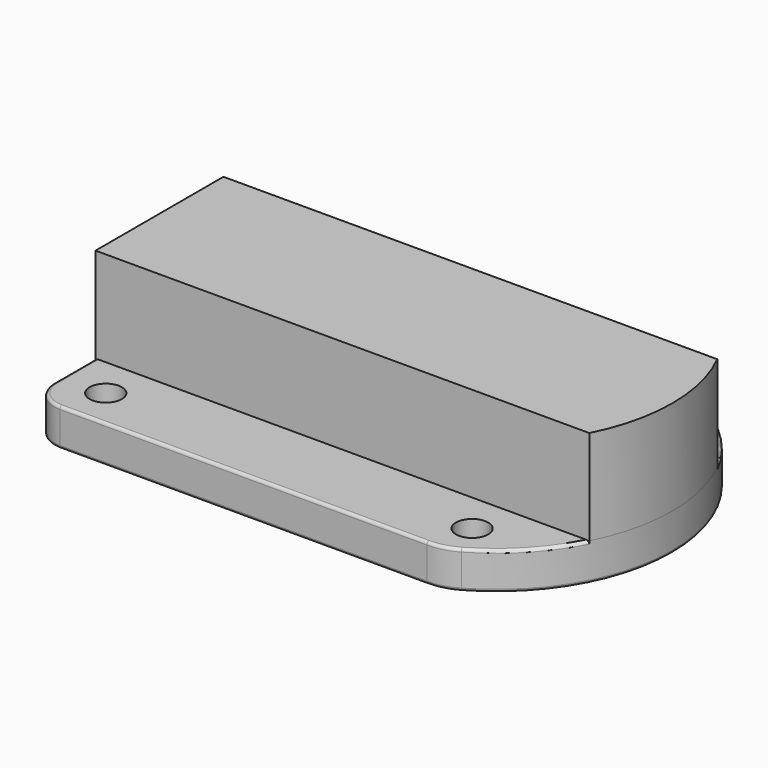
from build123d import *

# Parameters (mm, degrees)
F0_R         = 2.8
F1_DEPTH     = 6.5
F3_DEPTH     = 16.5
F4_T1_DEPTH  = 63.8184719387
F4_T3_DEPTH  = 45.8
F4_T5_DEPTH  = 9
F4_T7_DEPTH  = 9
F4_T10_ANGLE = 90
F4_T12_ANGLE = 120.4504110916
F4_T14_ANGLE = 90
F4_T16_ANGLE = 90
F4_T18_ANGLE = 29.7747944542
F4_T20_ANGLE = 29.7747944542
F4_T22_ANGLE = 29.7747944542
F4_T26_ANGLE = 35.5690080159
F4_T29_ANGLE = 90
F4_T33_ANGLE = 35.5690080159
F4_T36_ANGLE = 29.7747944542
F5_SIZE      = 1.56


# Not quite as in the source:
# - a fillet or chamfer that OpenCascade refuses, or shapes differently, is made with other operations: its cross-section is extruded or revolved along the edge and cut away or added


with BuildPart() as f1:
    # F0 (on Top) → F1 (new body)
    with BuildSketch(Plane.XY):
        with BuildLine():
            Line((-38.8770699501, 16.9000072956), (-38.8770699501, -28.8999927044))
            ThreePointArc((-38.8770699501, -28.8999927044), (-37.412603856, -32.4355266103), (-33.8770699501, -33.8999927044))
            Line((-33.8770699501, -33.8999927044), (29.9414019886, -33.8999927044))
            ThreePointArc((29.9414019886, -33.8999927044), (32.5106042183, -33.5643188528), (34.9073236464, -32.579832685))
            ThreePointArc((34.9073236464, -32.579832685), (50.3229300499, -5.9999927044), (34.9073236464, 20.5798472762))
            ThreePointArc((34.9073236464, 20.5798472762), (32.5106042183, 21.564333444), (29.9414019886, 21.9000072956))
            Line((29.9414019886, 21.9000072956), (-33.8770699501, 21.9000072956))
            ThreePointArc((-33.8770699501, 21.9000072956), (-37.412603856, 20.4355412015), (-38.8770699501, 16.9000072956))
        make_face()
        with Locations((-31.4170904458, -26.9999932498)):
            Circle(F0_R, mode=Mode.SUBTRACT)
        with Locations((32.2829300499, -26.9999927044)):
            Circle(F0_R, mode=Mode.SUBTRACT)
        with Locations((-31.4170904458, 15.0000071153)):
            Circle(F0_R, mode=Mode.SUBTRACT)
        with Locations((32.2829300499, 15.0000072956)):
            Circle(F0_R, mode=Mode.SUBTRACT)
    extrude(amount=F1_DEPTH)

    # F2 (on face) → F3 (join)
    with BuildSketch(Plane.XY.offset(6.5)):
        with BuildLine():
            Line((-38.8770699501, 7.9000072956), (-38.8770699501, -5.9999927044))
            Line((-38.8770699501, -5.9999927044), (-38.8770699501, -19.8999927044))
            Line((-38.8770699501, -19.8999927044), (46.9864613892, -19.8999927044))
            ThreePointArc((46.9864613892, -19.8999927044), (50.3229300499, -5.9999927044), (46.9864613892, 7.9000072956))
            Line((46.9864613892, 7.9000072956), (-38.8770699501, 7.9000072956))
        make_face()
    extrude(amount=F3_DEPTH)

    # F4: fillet of radius 0.5 on 18 edges, made by hand

    # F4_s2 → F4_t1 (cut)
    with BuildSketch(Plane.YZ.offset(-33.8770699501)):
        with BuildLine():
            ThreePointArc((21.9000072956, 0.5), (21.7535606862, 0.1464466094), (21.4000072956, 0))
            Line((21.4000072956, 0), (21.9000072956, 0))
            Line((21.9000072956, 0), (21.9000072956, 0.5))
        make_face()
        with BuildLine():
            ThreePointArc((21.9000072956, 6), (21.7535606862, 6.3535533906), (21.4000072956, 6.5))
            Line((21.4000072956, 6.5), (21.9000072956, 6.5))
            Line((21.9000072956, 6.5), (21.9000072956, 6))
        make_face()
        with BuildLine():
            ThreePointArc((-33.3999927044, 6.5), (-33.753546095, 6.3535533906), (-33.8999927044, 6))
            Line((-33.8999927044, 6), (-33.8999927044, 6.5))
            Line((-33.8999927044, 6.5), (-33.3999927044, 6.5))
        make_face()
        with BuildLine():
            ThreePointArc((-33.3999927044, 0), (-33.753546095, 0.1464466094), (-33.8999927044, 0.5))
            Line((-33.8999927044, 0.5), (-33.8999927044, 0))
            Line((-33.8999927044, 0), (-33.3999927044, 0))
        make_face()
    extrude(amount=F4_T1_DEPTH, mode=Mode.SUBTRACT)

    # F4_s4 → F4_t3 (cut)
    with BuildSketch(Plane.XZ.offset(-16.9000072956)):
        with BuildLine():
            ThreePointArc((-38.8770699501, 0.5), (-38.7306233407, 0.1464466094), (-38.3770699501, 0))
            Line((-38.3770699501, 0), (-38.8770699501, 0))
            Line((-38.8770699501, 0), (-38.8770699501, 0.5))
        make_face()
    extrude(amount=F4_T3_DEPTH, mode=Mode.SUBTRACT)

    # F4_s6 → F4_t5 (cut)
    with BuildSketch(Plane.XZ.offset(-16.9000072956)):
        with BuildLine():
            ThreePointArc((-38.8770699501, 6), (-38.7306233407, 6.3535533906), (-38.3770699501, 6.5))
            Line((-38.3770699501, 6.5), (-38.8770699501, 6.5))
            Line((-38.8770699501, 6.5), (-38.8770699501, 6))
        make_face()
    extrude(amount=F4_T5_DEPTH, mode=Mode.SUBTRACT)

    # F4_s8 → F4_t7 (cut)
    with BuildSketch(Plane.XZ.offset(19.8999927044)):
        with BuildLine():
            ThreePointArc((-38.8770699501, 6), (-38.7306233407, 6.3535533906), (-38.3770699501, 6.5))
            Line((-38.3770699501, 6.5), (-38.8770699501, 6.5))
            Line((-38.8770699501, 6.5), (-38.8770699501, 6))
        make_face()
    extrude(amount=F4_T7_DEPTH, mode=Mode.SUBTRACT)

    # F4_s9 → F4_t10 (revolve, cut)
    with BuildSketch(Plane.YZ.offset(-33.8770699501)):
        with BuildLine():
            ThreePointArc((21.9000072956, 0.5), (21.7535606862, 0.1464466094), (21.4000072956, 0))
            Line((21.4000072956, 0), (21.9000072956, 0))
            Line((21.9000072956, 0), (21.9000072956, 0.5))
        make_face()
    revolve(axis=Axis((-33.8770699501, 16.9000072956, 0), (0, 0, 1)), revolution_arc=F4_T10_ANGLE, mode=Mode.SUBTRACT)

    # F4_s11 → F4_t12 (revolve, cut)
    with BuildSketch(Plane(origin=(12.2560283734, 7.0119353437, 0), x_dir=(0, 0, 1), z_dir=(-0.8679839981, -0.4965921658, 0))):
        with BuildLine():
            ThreePointArc((0, -45.1134768811), (0.1464466094, -45.4670302717), (0.5, -45.6134768811))
            Line((0.5, -45.6134768811), (0, -45.6134768811))
            Line((0, -45.6134768811), (0, -45.1134768811))
        make_face()
    revolve(axis=Axis((19.7004300499, -5.9999927044, 0), (0, 0, 1)), revolution_arc=F4_T12_ANGLE, mode=Mode.SUBTRACT)

    # F4_s13 → F4_t14 (revolve, cut)
    with BuildSketch(Plane.YZ.offset(-33.8770699501)):
        with BuildLine():
            ThreePointArc((21.9000072956, 6), (21.7535606862, 6.3535533906), (21.4000072956, 6.5))
            Line((21.4000072956, 6.5), (21.9000072956, 6.5))
            Line((21.9000072956, 6.5), (21.9000072956, 6))
        make_face()
    revolve(axis=Axis((-33.8770699501, 16.9000072956, 6.5), (0, 0, 1)), revolution_arc=F4_T14_ANGLE, mode=Mode.SUBTRACT)

    # F4_s15 → F4_t16 (revolve, cut)
    with BuildSketch(Plane.XZ.offset(28.8999927044)):
        with BuildLine():
            ThreePointArc((-38.3770699501, 0), (-38.7306233407, 0.1464466094), (-38.8770699501, 0.5))
            Line((-38.8770699501, 0.5), (-38.8770699501, 0))
            Line((-38.8770699501, 0), (-38.3770699501, 0))
        make_face()
    revolve(axis=Axis((-33.8770699501, -28.8999927044, 0), (0, 0, 1)), revolution_arc=F4_T16_ANGLE, mode=Mode.SUBTRACT)

    # F4_s17 → F4_t18 (revolve, cut)
    with BuildSketch(Plane.YZ.offset(29.9414019886)):
        with BuildLine():
            ThreePointArc((-33.3999927044, 0), (-33.753546095, 0.1464466094), (-33.8999927044, 0.5))
            Line((-33.8999927044, 0.5), (-33.8999927044, 0))
            Line((-33.8999927044, 0), (-33.3999927044, 0))
        make_face()
    revolve(axis=Axis((29.9414019886, -23.8999927044, 0), (0, 0, 1)), revolution_arc=F4_T18_ANGLE, mode=Mode.SUBTRACT)

    # F4_s19 → F4_t20 (revolve, cut)
    with BuildSketch(Plane(origin=(17.4284307256, -9.9711770948, 0), x_dir=(0, 0, 1), z_dir=(0.8679839981, -0.4965921658, 0))):
        with BuildLine():
            ThreePointArc((0, -34.6976815693), (0.1464466094, -35.0512349599), (0.5, -35.1976815693))
            Line((0.5, -35.1976815693), (0, -35.1976815693))
            Line((0, -35.1976815693), (0, -34.6976815693))
        make_face()
    revolve(axis=Axis((29.9414019886, 11.9000072956, 0), (0, 0, 1)), revolution_arc=F4_T20_ANGLE, mode=Mode.SUBTRACT)

    # F4_s21 → F4_t22 (revolve, cut)
    with BuildSketch(Plane(origin=(17.4284307256, -9.9711770948, 0), x_dir=(0, 0, 1), z_dir=(0.8679839981, -0.4965921658, 0))):
        with BuildLine():
            ThreePointArc((6.5, -34.6976815693), (6.3535533906, -35.0512349599), (6, -35.1976815693))
            Line((6, -35.1976815693), (6.5, -35.1976815693))
            Line((6.5, -35.1976815693), (6.5, -34.6976815693))
        make_face()
    revolve(axis=Axis((29.9414019886, 11.9000072956, 6.5), (0, 0, 1)), revolution_arc=F4_T22_ANGLE, mode=Mode.SUBTRACT)


with BuildPart() as f4_tool24:
    # F4_s25 → F4_t26 (revolve)
    with BuildSketch(Plane(origin=(5.7033446243, -12.4249727464, 0), x_dir=(0, 0, 1), z_dir=(0.4171723997, -0.9088273703, 0))):
        with BuildLine():
            ThreePointArc((6.5, -45.5237586807), (6.3535533906, -45.8773120713), (6, -46.0237586807))
            Line((6, -46.0237586807), (6.5, -46.0237586807))
            Line((6.5, -46.0237586807), (6.5, -45.5237586807))
        make_face()
    revolve(axis=Axis((19.7004300499, -5.9999927044, 6.5), (0, 0, 1)), revolution_arc=F4_T26_ANGLE)

    split(bisect_by=Plane.XZ.offset(-7.9000072956), keep=Keep.BOTTOM)


with BuildPart() as f1_1:
    add(f1.part)

    # F4_t23: cut F4_tool24
    add(f4_tool24.part, mode=Mode.SUBTRACT)

    # F4_s28 → F4_t29 (revolve, cut)
    with BuildSketch(Plane.XZ.offset(28.8999927044)):
        with BuildLine():
            ThreePointArc((-38.8770699501, 6), (-38.7306233407, 6.3535533906), (-38.3770699501, 6.5))
            Line((-38.3770699501, 6.5), (-38.8770699501, 6.5))
            Line((-38.8770699501, 6.5), (-38.8770699501, 6))
        make_face()
    revolve(axis=Axis((-33.8770699501, -28.8999927044, 6.5), (0, 0, 1)), revolution_arc=F4_T29_ANGLE, mode=Mode.SUBTRACT)


with BuildPart() as f4_tool31:
    # F4_s32 → F4_t33 (revolve)
    with BuildSketch(Plane(origin=(12.2560283734, 7.0119353437, 0), x_dir=(0, 0, 1), z_dir=(-0.8679839981, -0.4965921658, 0))):
        with BuildLine():
            ThreePointArc((6.5, -45.1134768811), (6.3535533906, -45.4670302717), (6, -45.6134768811))
            Line((6, -45.6134768811), (6.5, -45.6134768811))
            Line((6.5, -45.6134768811), (6.5, -45.1134768811))
        make_face()
    revolve(axis=Axis((19.7004300499, -5.9999927044, 6.5), (0, 0, 1)), revolution_arc=F4_T33_ANGLE)

    split(bisect_by=Plane.XZ.offset(19.8999927044), keep=Keep.TOP)


with BuildPart() as f1_2:
    add(f1_1.part)

    # F4_t30: cut F4_tool31
    add(f4_tool31.part, mode=Mode.SUBTRACT)

    # F4_s35 → F4_t36 (revolve, cut)
    with BuildSketch(Plane.YZ.offset(29.9414019886)):
        with BuildLine():
            ThreePointArc((-33.3999927044, 6.5), (-33.753546095, 6.3535533906), (-33.8999927044, 6))
            Line((-33.8999927044, 6), (-33.8999927044, 6.5))
            Line((-33.8999927044, 6.5), (-33.3999927044, 6.5))
        make_face()
    revolve(axis=Axis((29.9414019886, -23.8999927044, 6.5), (0, 0, 1)), revolution_arc=F4_T36_ANGLE, mode=Mode.SUBTRACT)

    # F5
    f5_edges = [f1_2.edges().sort_by_distance(p)[0] for p in [
        (-34.21709, 15.000007, 0),
        (-34.21709, -26.999993, 0),
        (29.48293, -26.999993, 0),
        (29.48293, 15.000007, 0),
    ]]
    chamfer(f5_edges, length=F5_SIZE)


solid = f1_2.part
